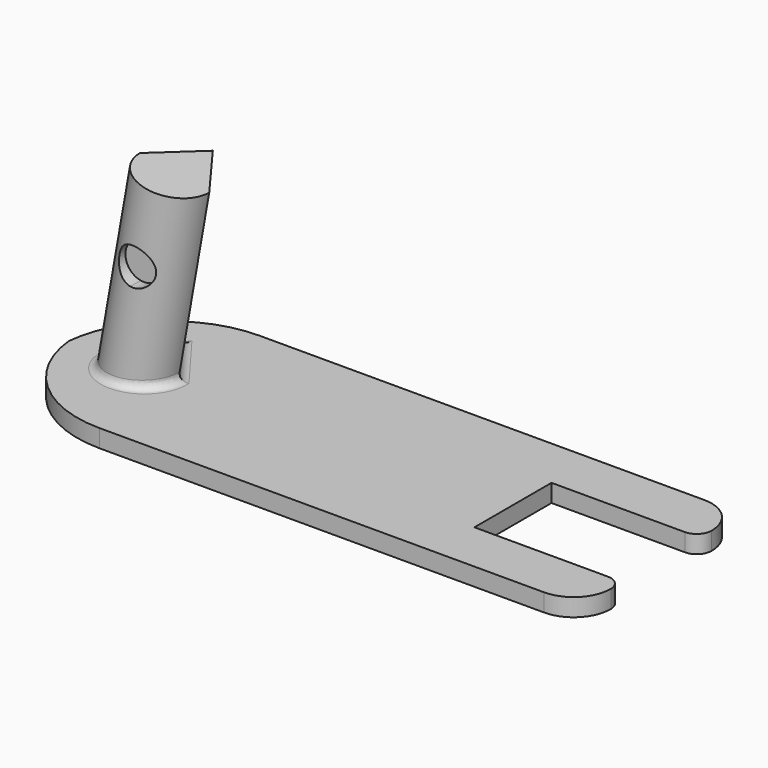
from build123d import *

# Parameters (mm, degrees)
F1_DEPTH      = 2.4
F4_DEPTH      = 25
F4_DEPTH_BACK = 1
F5_R          = 5
F6_T1_DEPTH   = 77.4
F7_R          = 1
F8_R          = 1.99999
F10_START     = 3
F10_DEPTH     = 22


# Not quite as in the source:
# - a fillet or chamfer that OpenCascade refuses, or shapes differently, is made with other operations: its cross-section is extruded or revolved along the edge and cut away or added
# - a fillet or chamfer is up to 0.001 mm smaller than in the source, because OpenCascade refuses the exact size


with BuildPart() as f1:
    # F0 (on Top) → F1 (new body)
    with BuildSketch(Plane.XY):
        Polygon((70, 13.5), (-10, 13.5), (-10, -13.5), (70, -13.5), (70, -6.5), (50, -6.5), (50, 6.5), (70, 6.5), align=None)
        with BuildLine():
            ThreePointArc((4.75, 0), (0, -4.75), (-4.75, 0))
            Line((-4.75, 0), (0, 6.45))
            Line((0, 6.45), (4.75, 0))
        make_face(mode=Mode.SUBTRACT)
        with BuildLine():
            Line((0, 6.45), (-4.75, 0))
            ThreePointArc((-4.75, 0), (0, -4.75), (4.75, 0))
            Line((4.75, 0), (0, 6.45))
        make_face()
    extrude(amount=-F1_DEPTH)

    # F3 (on line) → F4 (join, two sides)
    with BuildSketch(Plane(origin=(0, 0, 0), x_dir=(0.984807753, 0, -0.1736481777), z_dir=(-0.1736481777, 0, -0.984807753))) as f4_sk:
        with BuildLine():
            ThreePointArc((4.75, 0), (0, 4.75), (-4.75, 0))
            Line((-4.75, 0), (0, -6.45))
            Line((0, -6.45), (4.75, 0))
        make_face()
    extrude(amount=-F4_DEPTH)
    extrude(f4_sk.sketch, amount=F4_DEPTH_BACK)

    # F5
    f5_edges = [f1.edges().sort_by_distance(p)[0] for p in [
        (70, -13.5, -1.2),
        (70, 13.5, -1.2),
    ]]
    fillet(f5_edges, radius=F5_R)

    # F6: fillet of radius 15 on 2 edges, made by hand

    # F6_s2 → F6_t1 (cut)
    with BuildSketch(Plane.XY.offset(-39.9)):
        with BuildLine():
            ThreePointArc((-10, 1.5), (-5.6066017178, -9.1066017178), (5, -13.5))
            Line((5, -13.5), (-10, -13.5))
            Line((-10, -13.5), (-10, 1.5))
        make_face()
        with BuildLine():
            ThreePointArc((5, 13.5), (-5.6066017178, 9.1066017178), (-10, -1.5))
            Line((-10, -1.5), (-10, 13.5))
            Line((-10, 13.5), (5, 13.5))
        make_face()
    extrude(amount=F6_T1_DEPTH, mode=Mode.SUBTRACT)

    # F7
    f7_edges = [f1.edges().sort_by_distance(p)[0] for p in [
        (0, -4.75, 0),
        (-2.411638, 3.225, 0),
        (2.411638, 3.225, 0),
    ]]
    fillet(f7_edges, radius=F7_R)

    # F8 (radius 2 in the source; OpenCascade refuses exactly that, so slightly less here)
    f8_edges = [f1.edges().sort_by_distance(p)[0] for p in [
        (70, 6.5, -1.2),
        (70, -6.5, -1.2),
    ]]
    fillet(f8_edges, radius=F8_R)

    # F9 (on Front) → F10 (cut)
    with BuildSketch(Plane.XZ.offset(F10_START)):
        with BuildLine():
            ThreePointArc((2.1757445863, 12.3392607162), (4.2168340546, 12.8861689909), (5.1098650304, 14.8012800987))
            ThreePointArc((5.1098650304, 14.8012800987), (4.5249761382, 16.4082491229), (3.0439854746, 17.2632994812))
            Line((3.0439854746, 17.2632994812), (2.1757445863, 12.3392607162))
        make_face()
        with BuildLine():
            Line((2.1757445863, 12.3392607162), (3.0439854746, 17.2632994812))
            ThreePointArc((3.0439854746, 17.2632994812), (0.1478456479, 15.2354005429), (2.1757445863, 12.3392607162))
        make_face()
    extrude(amount=F10_DEPTH, mode=Mode.SUBTRACT)


solid = f1.part
